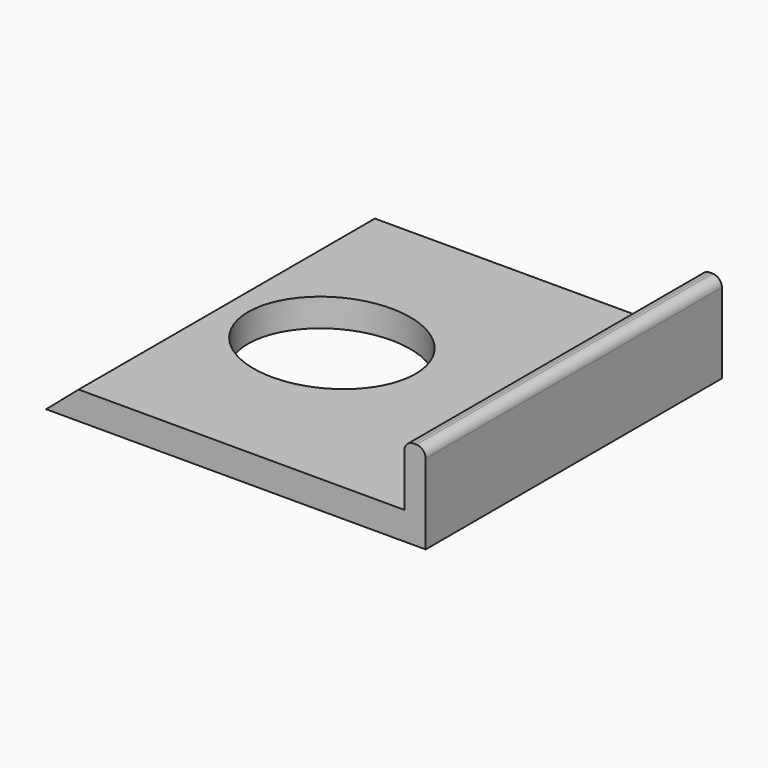
from build123d import *

# Parameters (mm, degrees)
F0_W     = 38.5
F0_H     = 39.8
F0_W_2   = 2.3
F1_DEPTH = 3
F2_DEPTH = 9.6
F3_R     = 1
F4_SIZE2 = 2.99999
F4_SIZE  = 3.49999


# Not quite as in the source:
# - a fillet or chamfer is up to 0.001 mm smaller than in the source, because OpenCascade refuses the exact size


with BuildPart() as f1:
    # F0 (on Top) → F1 (new body)
    with BuildSketch(Plane.XY):
        with Locations((-1.15, 0)):
            Rectangle(F0_W, F0_H)
        with BuildLine():
            add(Edge.make_bspline(
                [(3.4, 0), (3.4, 13.8564064606), (-10.1, 6.9282032303), (-23.6, 0), (-10.1, -6.9282032303), (3.4, -13.8564064606), (3.4, 0)],
                knots=[0, 0, 0, 2.0943951024, 2.0943951024, 4.1887902048, 4.1887902048, 6.2831853072, 6.2831853072, 6.2831853072], degree=2, weights=[1, 0.5, 1, 0.5, 1, 0.5, 1]))
        make_face(mode=Mode.SUBTRACT)
        with Locations((19.25, 0)):
            Rectangle(F0_W_2, F0_H)
    extrude(amount=F1_DEPTH)

    # F0 (on Top) → F2 (join)
    with BuildSketch(Plane.XY):
        with Locations((19.25, 0)):
            Rectangle(F0_W_2, F0_H)
    extrude(amount=F2_DEPTH)

    # F3
    f3_edges = [f1.edges().sort_by_distance(p)[0] for p in [
        (18.1, 0, 9.6),
        (20.4, 0, 9.6),
    ]]
    fillet(f3_edges, radius=F3_R)

    # F4 (size 3.5 and 3 in the source; OpenCascade refuses exactly that, so slightly less here)
    f4_edges = [f1.edges().sort_by_distance(p)[0] for p in [
        (-20.4, 0, 3),
    ]]
    f4_side = f1.faces().sort_by_distance((-1.15, 19.346259, 3))[0]
    chamfer(f4_edges, length=F4_SIZE, length2=F4_SIZE2, reference=f4_side)


solid = f1.part
